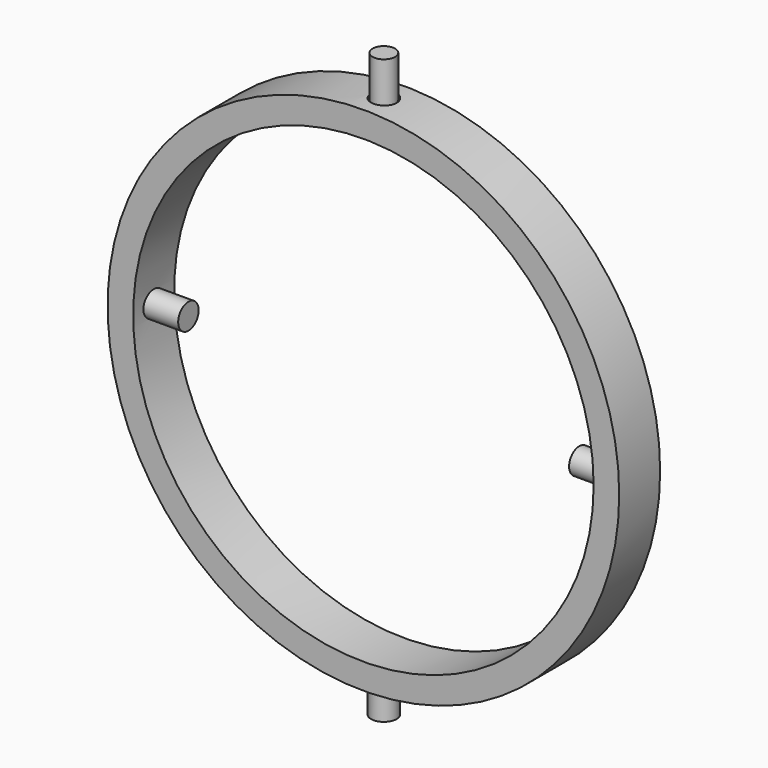
from build123d import *

# Parameters (mm, degrees)
F0_R      = 25
F0_R_2    = 22.5
F1_DEPTH  = 5
F3_R      = 1.25
F4_DEPTH  = 3.8
F6_R      = 1.25
F7_DEPTH  = 3.4
F8_R      = 1.25
F9_DEPTH  = 0.25
F10_R     = 1.25
F11_DEPTH = 0.25
F13_R     = 1.25
F13_R_2   = 1.1
F14_DEPTH = 25
F16_R     = 1.25
F17_DEPTH = 4.4


# Not quite as in the source:
# - a pattern or mirror of a feature is missing from the dataset's text; its kind, count and spacing are read off the source's solid


with BuildPart() as f1:
    # F0 (on Front) → F1 (new body)
    with BuildSketch(Plane.XZ):
        Circle(F0_R)
        Circle(F0_R_2, mode=Mode.SUBTRACT)
    extrude(amount=F1_DEPTH)

    # F3 (on offset) → F4 (join)
    with BuildSketch(Plane.XY.offset(24.83)):
        with Locations((0, -2.5)):
            Circle(F3_R)
    extrude(amount=F4_DEPTH)

    # F6 (on offset) → F7 (join)
    with BuildSketch(Plane.XY.offset(-24.39)):
        with Locations((0, -2.5)):
            Circle(F6_R)
    extrude(amount=-F7_DEPTH)

    # F8 (on face) → F9 (join)
    with BuildSketch(Plane(origin=(0, 0, -27.79), x_dir=(1, 0, 0), z_dir=(0, 0, -1))):
        with Locations((0, 2.5)):
            Circle(F8_R)
    extrude(amount=F9_DEPTH)

    # F10 (on face) → F11 (join)
    with BuildSketch(Plane.XY.offset(28.63)):
        with Locations((0, -2.5)):
            Circle(F10_R)
    extrude(amount=F11_DEPTH)

    # F13 (on offset) → F14 (cut)
    with BuildSketch(Plane.XY.offset(24.83)):
        with Locations((0, -2.5)):
            Circle(F13_R)
        with Locations((0, -2.5)):
            Circle(F13_R_2, mode=Mode.SUBTRACT)
    extrude(amount=F14_DEPTH, mode=Mode.SUBTRACT)

    # F16 (on offset) → F17 (join)
    with BuildSketch(Plane.YZ.offset(23.5)):
        with Locations((-2.5, 0)):
            Circle(F16_R)
    f17 = extrude(amount=-F17_DEPTH)

    # F17_copies: F17 across plane
    add(f17.mirror(Plane(origin=(0, 0, 0), x_dir=(0, 0, -1), z_dir=(-1, 0, 0))))


solid = f1.part
